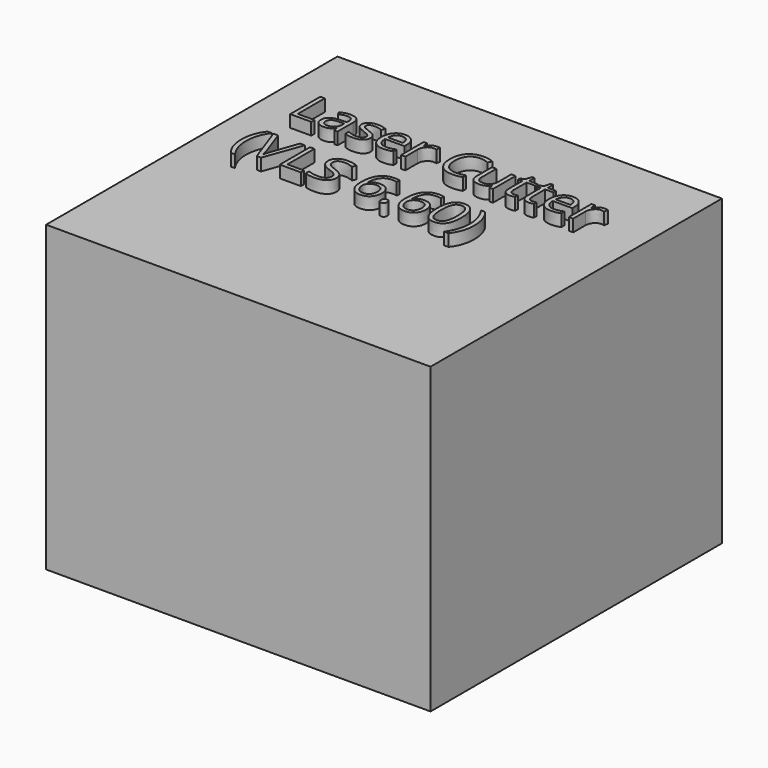
from build123d import *

# Parameters (mm, degrees)
F0_W         = 965.2
F0_H         = 914.4
F1_DEPTH     = 762
F2_TEXT_SIZE = 132.4749409176
F3_DEPTH     = 30.48


# Not quite as in the source:
# - Text() gives the source's letters only with a copy of the font that has no kerning and outlines rounded to 1/6400 em; it was checked with that copy


with BuildPart() as f1:
    # F0 (on Top) → F1 (new body)
    with BuildSketch(Plane.XY):
        Rectangle(F0_W, F0_H)
    extrude(amount=F1_DEPTH)

    # F2 (on face) → F3 (join)
    with BuildSketch(Plane.XY.offset(762)):
        with Locations((-378.6026901163, 162.7688786409)):
            Text('Laser Cutter', F2_TEXT_SIZE, font='Open Sans', text_align=(TextAlign.LEFT, TextAlign.BOTTOM))
        with Locations((-378.6026901163, -17.3970410071)):
            Text('(VLS 6.60)', F2_TEXT_SIZE, font='Open Sans', text_align=(TextAlign.LEFT, TextAlign.BOTTOM))
    extrude(amount=F3_DEPTH)


solid = f1.part
